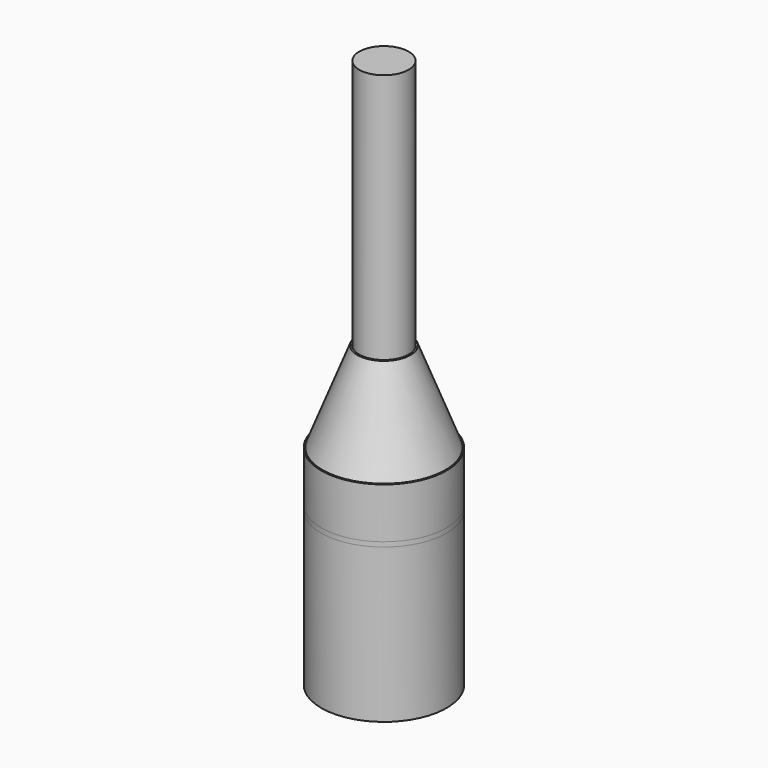
from build123d import *

# Parameters (mm, degrees)
F0_W  = 38.1
F0_H  = 127
F4_W  = 15.1131534949
F4_H  = 210.3794142604
F6_W  = 28.5528358072
F6_H  = 138.149574399
F8_W  = 14.9974487722
F8_H  = 254
F12_W = 29.4399373233
F12_H = 1.5613138676
F14_W = 38.1
F14_H = 2.8206296265
F16_W = 21.6601658612
F16_H = 20.3340332955


# Not quite as in the source:
# - a feature of the source that left no trace in its solid (it failed there, or was rolled back) is left out


with BuildPart() as f1:
    # F0 (on Front) → F1 (revolve)
    with BuildSketch(Plane.XZ):
        with Locations((-19.05, 4.4871026874)):
            Rectangle(F0_W, F0_H)
    revolve(axis=Axis((0, 0, 4.4871026874), (0, 0, -1)))

    # F2 (on Front) → F3 (revolve)
    with BuildSketch(Plane.XZ):
        Polygon((-37.352733314, 68.0748075247), (0, 67.8537860513), (0, 122.6672679186), (-16.1346122622, 122.6672679186), align=None)
    revolve(axis=Axis((0, 0, 95.2605269849), (0, 0, 1)))

    # F4 (on Front) → F5 (revolve, cut)
    with BuildSketch(Plane.XZ):
        with Locations((-7.5565767474, 30.3173996508)):
            Rectangle(F4_W, F4_H)
    revolve(axis=Axis((0, 0, 30.3173996508), (0, 0, 1)), mode=Mode.SUBTRACT)

    # F6 (on Front) → F7 (revolve, cut)
    with BuildSketch(Plane.XZ):
        with Locations((-14.2764179036, -1.1372193694)):
            Rectangle(F6_W, F6_H)
    revolve(axis=Axis((0, 0, -1.1372193694), (0, 0, 1)), mode=Mode.SUBTRACT)

    # F14 (on Front) → F15 (revolve)
    with BuildSketch(Plane.XZ):
        with Locations((-19.05, 35.9340105206)):
            Rectangle(F14_W, F14_H)
    revolve(axis=Axis((0, 0, 35.9340105206), (0, 0, 1)))

    # F16 (on Front) → F17 (revolve, cut)
    with BuildSketch(Plane.XZ):
        with Locations((-10.8300829306, 32.0482039824)):
            Rectangle(F16_W, F16_H)
    revolve(axis=Axis((0, 0, 32.0482039824), (0, 0, -1)), mode=Mode.SUBTRACT)


with BuildPart() as f9:
    # F8 (on Front) → F9 (revolve)
    with BuildSketch(Plane.XZ):
        with Locations((-7.4987243861, 147.9263339639)):
            Rectangle(F8_W, F8_H)
    revolve(axis=Axis((0, 0, 147.9263339639), (0, 0, 1)))

    # F12 (on Front) → F13 (revolve)
    with BuildSketch(Plane.XZ):
        with Locations((-14.7199686617, 46.5829521418)):
            Rectangle(F12_W, F12_H)
    revolve(axis=Axis((0, 0, 46.5829521418), (0, 0, 1)))


solid = Compound([f1.part, f9.part])
